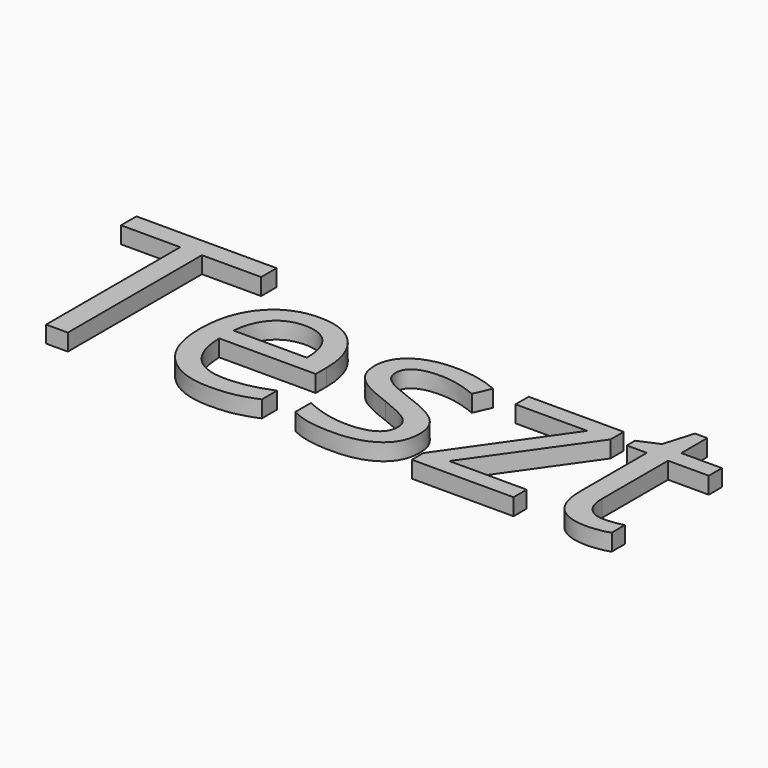
from build123d import *

# Parameters (mm, degrees)
F0_TEXT_SIZE = 15.6283430946
F1_DEPTH     = 1


# Not quite as in the source:
# - Text() gives the source's letters only with a copy of the font that has no kerning and outlines rounded to 1/6400 em; it was checked with that copy


with BuildPart() as f1:
    # F0 (on Top) → F1 (new body)
    with BuildSketch(Plane.XY):
        with Locations((-13.7529408132, 0)):
            Text('Teszt', F0_TEXT_SIZE, font='Open Sans', text_align=(TextAlign.LEFT, TextAlign.BOTTOM))
    extrude(amount=F1_DEPTH)


solid = f1.part
